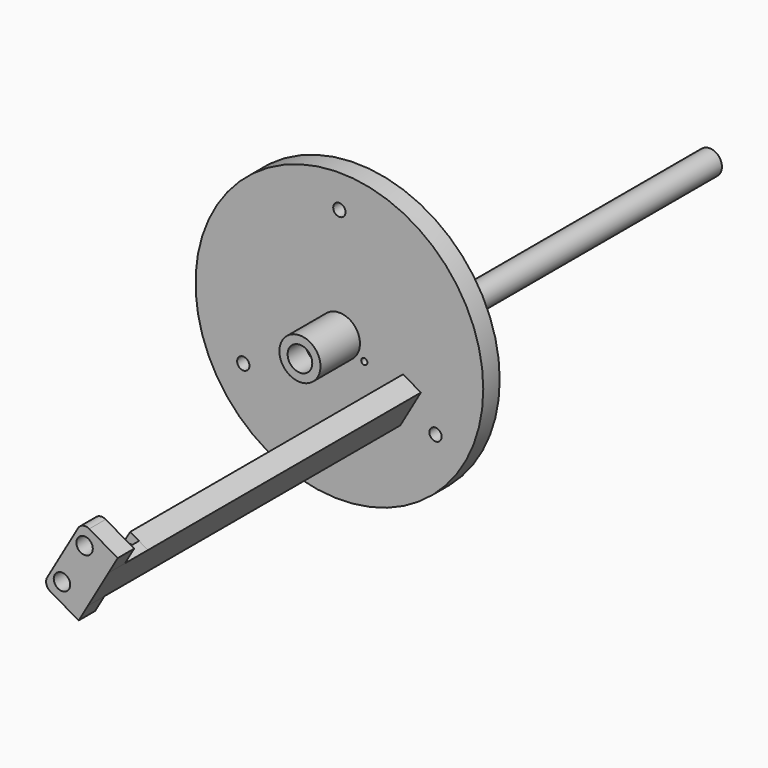
from build123d import *

# Parameters (mm, degrees)
F0_R      = 35
F1_DEPTH  = 5
F2_R      = 5
F2_R_2    = 3
F3_DEPTH  = 12
F5_DEPTH  = 83
F7_D      = 3
F7_DEPTH  = 6
F7_TIP    = 0.9012909285
F9_DEPTH  = 83
F10_R     = 3
F11_DEPTH = 6.5
F13_DEPTH = 7
F15_DEPTH = 5
F17_D     = 4
F17_DEPTH = 10
F17_TIP   = 1.2017212381
F19_D     = 1.5
F19_DEPTH = 10
F19_TIP   = 0.4506454643
F20_R     = 3
F20_R_2   = 1.5
F21_DEPTH = 100


# Not quite as in the source:
# - a feature names something its author has since deleted; it is built from what else it names


with BuildPart() as f1:
    # F0 (on Front) → F1 (new body)
    with BuildSketch(Plane.XZ):
        Circle(F0_R)
    extrude(amount=F1_DEPTH)

    # F2 (on face) → F3 (join)
    with BuildSketch(Plane.XZ.offset(5)):
        Circle(F2_R)
        Circle(F2_R_2, mode=Mode.SUBTRACT)
    extrude(amount=F3_DEPTH)

    # F4 (on face) → F5 (join)
    with BuildSketch(Plane.XZ.offset(5)):
        Polygon((14.8205080757, -14.3301270189), (19.8205080757, -5.6698729811), (15.4903810568, -3.1698729811), (10.4903810568, -11.8301270189), align=None)
    extrude(amount=F5_DEPTH)

    # F7
    with Locations(Plane(origin=(0, 0, 0), x_dir=(-1, 0, 0), z_dir=(0, 1, 0))):
        with Locations((0, 27), (-23.3826859022, -13.5), (23.3826859022, -13.5)):
            Hole(F7_D / 2, depth=F7_DEPTH)
            with Locations((0, 0, -(F7_DEPTH + F7_TIP / 2))):  # 118° drill point
                Cone(0, F7_D / 2, F7_TIP, mode=Mode.SUBTRACT)

    # F8 (on face) → F9 (cut, through all)
    with BuildSketch(Plane.XZ.offset(88)):
        with BuildLine():
            Line((13.9903810568, -5.7679491924), (11.9903810568, -9.2320508076))
            Line((11.9903810568, -9.2320508076), (13.0007440278, -10.9820508076))
            ThreePointArc((13.0007440278, -10.9820508076), (13.4337567297, -11.2320508076), (13.8667694316, -10.9820508076))
            Line((13.8667694316, -10.9820508076), (16.4441197008, -6.5179491924))
            ThreePointArc((16.4441197008, -6.5179491924), (16.4441197008, -6.0179491924), (16.0111069989, -5.7679491924))
            Line((16.0111069989, -5.7679491924), (13.9903810568, -5.7679491924))
        make_face()
    extrude(amount=-F9_DEPTH, mode=Mode.SUBTRACT)

    # F10 (on face) → F11 (join)
    with BuildSketch(Plane.XZ.offset(5)):
        Circle(F10_R)
    extrude(amount=F11_DEPTH)

    # F12 (on face) → F13 (join)
    with BuildSketch(Plane.XZ.offset(88)):
        Polygon((12.6554445662, -13.0801270189), (14.8205080757, -14.3301270189), (19.8205080757, -5.6698729811), (17.6554445662, -4.4198729811), align=None)
    extrude(amount=F13_DEPTH)

    # F14 (on face) → F15 (join)
    with BuildSketch(Plane.XZ.offset(95)):
        with BuildLine():
            Line((5.6423048454, -14.227241336), (12.5705080757, -18.227241336))
            Line((12.5705080757, -18.227241336), (14.8205080757, -14.3301270189))
            Line((14.8205080757, -14.3301270189), (12.6554445662, -13.0801270189))
            Line((12.6554445662, -13.0801270189), (17.6554445662, -4.4198729811))
            Line((17.6554445662, -4.4198729811), (19.8205080757, -5.6698729811))
            Line((19.8205080757, -5.6698729811), (22.0705080757, -1.772758664))
            Line((22.0705080757, -1.772758664), (15.1423048454, 2.227241336))
            ThreePointArc((15.1423048454, 2.227241336), (13.6246667552, 2.427042181), (12.4102540378, 1.4951905284))
            Line((12.4102540378, 1.4951905284), (4.9102540378, -11.4951905284))
            ThreePointArc((4.9102540378, -11.4951905284), (4.7104531928, -13.0128286186), (5.6423048454, -14.227241336))
        make_face()
        Polygon((12.6554445662, -13.0801270189), (14.8205080757, -14.3301270189), (19.8205080757, -5.6698729811), (17.6554445662, -4.4198729811), align=None)
    extrude(amount=F15_DEPTH)

    # F17
    with Locations(Plane.XZ.offset(100)):
        with Locations((14.0083302492, -1.7368602792), (8.5083302492, -11.2631397208)):
            Hole(F17_D / 2, depth=F17_DEPTH)
            with Locations((0, 0, -(F17_DEPTH + F17_TIP / 2))):  # 118° drill point
                Cone(0, F17_D / 2, F17_TIP, mode=Mode.SUBTRACT)

    # F19
    with Locations(Plane.XZ.offset(5)):
        with Locations((6.0621778265, -3.5)):
            Hole(F19_D / 2, depth=F19_DEPTH)
            with Locations((0, 0, -(F19_DEPTH + F19_TIP / 2))):  # 118° drill point
                Cone(0, F19_D / 2, F19_TIP, mode=Mode.SUBTRACT)

    # F20 (on face) → F21 (join)
    with BuildSketch(Plane(origin=(0, 0, 0), x_dir=(-1, 0, 0), z_dir=(0, 1, 0))):
        with Locations((-6.0621778265, -3.5)):
            Circle(F20_R)
        with Locations((-6.0621778265, -3.5)):
            Circle(F20_R_2, mode=Mode.SUBTRACT)
    extrude(amount=F21_DEPTH)


solid = f1.part
